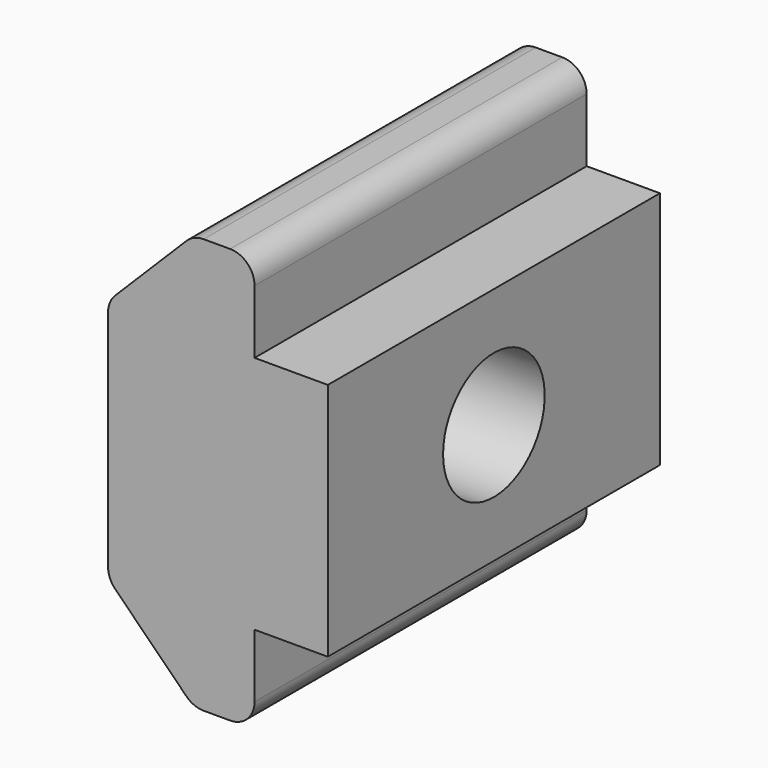
from build123d import *

# Parameters (mm, degrees)
F1_DEPTH = 17
F2_R     = 2.6
F3_DEPTH = 3.4
F4_DEPTH = 9.001


# Not quite as in the source:
# - ends of sketch curves that miss each other by under 0.0002 mm in the source are joined


with BuildPart() as f1:
    # F0 (on Front) → F1 (new body)
    with BuildSketch(Plane.XZ):
        with BuildLine():
            ThreePointArc((-8.4332967812, 5.0428927812), (-8.6500695325, 4.7184694324), (-8.72619, 4.335786))
            Line((-8.72619, 4.335786), (-8.72619, -4.835786))
            ThreePointArc((-8.72619, -4.835786), (-8.6500695325, -5.2184694324), (-8.4332967812, -5.5428927812))
            Line((-8.4332967812, -5.5428927812), (-5.519083, -8.457107))
            ThreePointArc((-5.519083, -8.457107), (-5.1946594324, -8.6738795325), (-4.811976, -8.75))
            Line((-4.811976, -8.75), (-3.72619, -8.75))
            ThreePointArc((-3.72619, -8.75), (-3.0190832188, -8.4571067812), (-2.72619, -7.75))
            Line((-2.72619, -7.75), (-2.72619, -5.15))
            Line((-2.72619, -5.15), (0.27381, -5.15))
            Line((0.27381, -5.15), (0.27381, 4.65))
            Line((0.27381, 4.65), (-2.72619, 4.65))
            Line((-2.72619, 4.65), (-2.72619, 7.25))
            ThreePointArc((-2.72619, 7.25), (-3.0190832188, 7.9571067812), (-3.72619, 8.25))
            Line((-3.72619, 8.25), (-4.811976, 8.25))
            ThreePointArc((-4.811976, 8.25), (-5.1946594324, 8.1738795325), (-5.5190827812, 7.9571067812))
            Line((-5.5190827812, 7.9571067812), (-8.4332967812, 5.0428927812))
        make_face()
    extrude(amount=-F1_DEPTH)

    # F2 (on face) → F3 (cut)
    with BuildSketch(Plane(origin=(-8.72619, 0, 0), x_dir=(0, -1, 0), z_dir=(-1, 0, 0))):
        Polygon((-11.6258979104, -4.835786), (-5.3741020896, -4.835786), (-2.7264973081, -0.25), (-5.3741020896, 4.335786), (-11.6258979104, 4.335786), (-14.2735026919, -0.25), align=None)
        with Locations((-8.5, -0.25)):
            Circle(F2_R, mode=Mode.SUBTRACT)
        with Locations((-8.5, -0.25)):
            Circle(F2_R)
    extrude(amount=-F3_DEPTH, mode=Mode.SUBTRACT)

    # F2 (on face) → F4 (cut, through all)
    with BuildSketch(Plane(origin=(-8.72619, 0, 0), x_dir=(0, -1, 0), z_dir=(-1, 0, 0))):
        with Locations((-8.5, -0.25)):
            Circle(F2_R)
    extrude(amount=-F4_DEPTH, mode=Mode.SUBTRACT)


solid = f1.part
